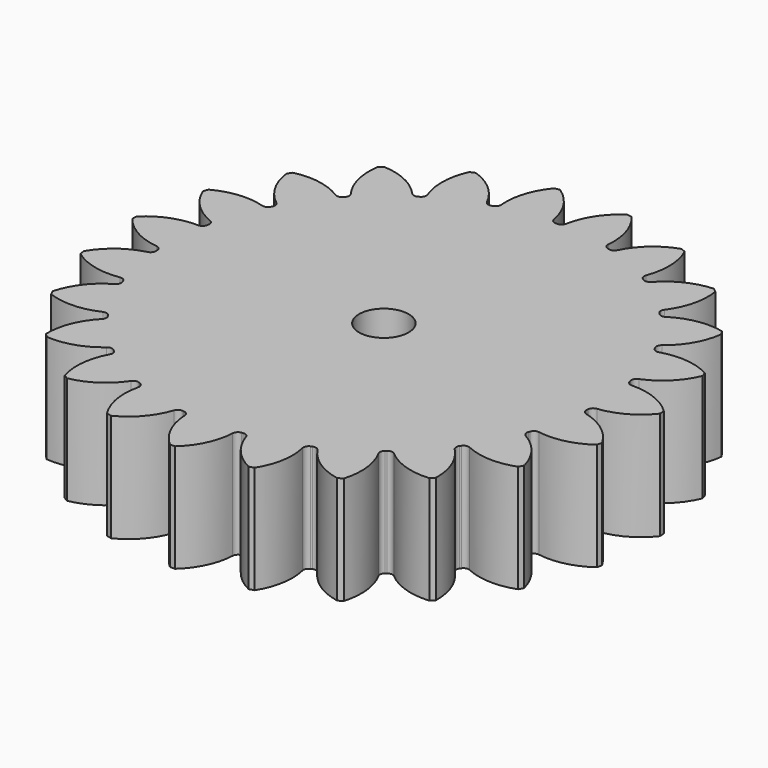
from build123d import *

# Parameters (mm, degrees)
F0_R     = 12.25
F0_R_2   = 1.15
F1_DEPTH = 5
F3_DEPTH = 25
F4_COUNT = 23


with BuildPart() as f1:
    # F0 (on Top) → F1 (new body)
    with BuildSketch(Plane.XY):
        Circle(F0_R)
        Circle(F0_R_2, mode=Mode.SUBTRACT)
    extrude(amount=F1_DEPTH)

    # F2 (on face) → F3 (cut)
    with BuildSketch(Plane.XY.offset(5)):
        with BuildLine():
            ThreePointArc((0.2804438166, 10.2051242801), (0.7191015118, 11.3062536781), (1.55, 12.1515431119))
            ThreePointArc((1.55, 12.1515431119), (0, 12.25), (-1.55, 12.1515431119))
            ThreePointArc((-1.55, 12.1515431119), (-0.7191015118, 11.3062536781), (-0.2804438166, 10.2051242801))
            ThreePointArc((-0.2804438166, 10.2051242801), (-0.1943199055, 10.057703465), (-0.0336525573, 9.9999433751))
            ThreePointArc((-0.0336525573, 9.9999433751), (0, 10), (0.0336525573, 9.9999433751))
            ThreePointArc((0.0336525573, 9.9999433751), (0.1943199055, 10.057703465), (0.2804438166, 10.2051242801))
        make_face()
    f3 = extrude(amount=-F3_DEPTH, mode=Mode.SUBTRACT)

    # F4: F3 ×23 about axis
    f4_axis = Axis((0, 0, 0), (0, 0, -1))
    for i in range(1, F4_COUNT):
        add(f3.rotate(f4_axis, i * 360 / F4_COUNT), mode=Mode.SUBTRACT)


solid = f1.part
